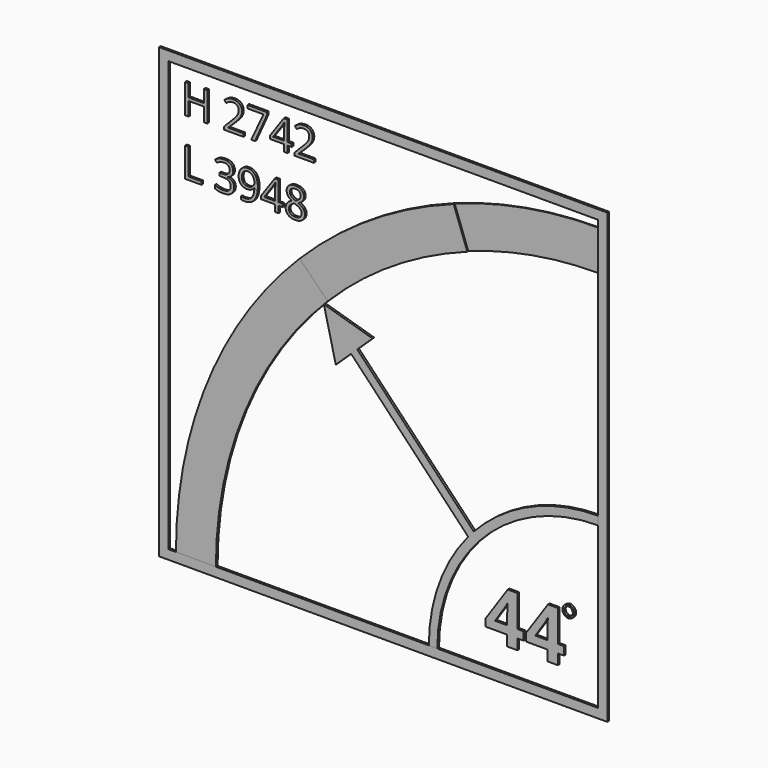
from build123d import *

# Parameters (mm, degrees)
F1_DEPTH       = 0.5
F3_DEPTH       = 0.5
F5_DEPTH       = 0.2
F6_W           = 106
F6_H           = 106
F6_W_2         = 101.6
F6_H_2         = 101.6
F7_DEPTH       = 0.5
F8_R           = 1.428350153
F8_R_2         = 1.0395037254
F8_TEXT_SIZE   = 16.6666666667
F8_TEXT_SIZE_2 = 9.7222222222
F9_DEPTH       = 0.5


# Not quite as in the source:
# - Text() gives the source's letters only with a copy of the font that has no kerning and outlines rounded to 1/6400 em; it was checked with that copy


with BuildPart() as f1:
    # F0 (on Front) → F1 (new body)
    with BuildSketch(Plane.XZ):
        with BuildLine():
            ThreePointArc((-19.7674013949, 19.7674013949), (-41.4007531902, -12.6091975676), (-48.9973761141, -50.8))
            Line((-48.9973761141, -50.8), (-39.5521000028, -50.8))
            ThreePointArc((-39.5521000028, -50.8), (-32.674455912, -16.2237482495), (-13.0885826064, 13.0885826064))
            Line((-13.0885826064, 13.0885826064), (-19.7674013949, 19.7674013949))
        make_face()
    extrude(amount=F1_DEPTH)


with BuildPart() as f3:
    # F2 (on Front) → F3 (new body)
    with BuildSketch(Plane.XZ):
        with BuildLine():
            ThreePointArc((16.6672871179, 42.9788579082), (-2.8210911002, 33.3682533292), (-19.7674013949, 19.7674013949))
            Line((-19.7674013949, 19.7674013949), (-13.0885826064, 13.0885826064))
            ThreePointArc((-13.0885826064, 13.0885826064), (2.2538520552, 25.4021882536), (19.8977618073, 34.1032016451))
            Line((19.8977618073, 34.1032016451), (16.6672871179, 42.9788579082))
        make_face()
    extrude(amount=F3_DEPTH)


with BuildPart() as f5:
    # F4 (on Front) → F5 (new body)
    with BuildSketch(Plane.XZ):
        with BuildLine():
            ThreePointArc((50.8, 48.9973761141), (33.4703675018, 47.4812297275), (16.6672871179, 42.9788579082))
            Line((16.6672871179, 42.9788579082), (19.8977960102, 34.1031076732))
            ThreePointArc((19.8977960102, 34.1031076732), (35.1105398514, 38.1793501002), (50.8, 39.552))
            Line((50.8, 39.552), (50.8, 48.9973761141))
        make_face()
    extrude(amount=F5_DEPTH)


with BuildPart() as f7:
    # F6 (on Front) → F7 (new body)
    with BuildSketch(Plane.XZ):
        Rectangle(F6_W, F6_H)
        Rectangle(F6_W_2, F6_H_2, mode=Mode.SUBTRACT)
    extrude(amount=F7_DEPTH)


with BuildPart() as f9:
    # F8 (on Front) → F9 (new body)
    with BuildSketch(Plane.XZ):
        with BuildLine():
            Line((21.4240073654, -23.6513157458), (-6.1287743468, 5.3071468295))
            Line((-6.1287743468, 5.3071468295), (-2.5064167724, 8.7536705278))
            Line((-2.5064167724, 8.7536705278), (-14.0167108476, 12.1467709243))
            Line((-14.0167108476, 12.1467709243), (-11.200074951, 0.4820136519))
            Line((-11.200074951, 0.4820136519), (-7.5777173766, 3.9285373502))
            Line((-7.5777173766, 3.9285373502), (20.098580007, -25.1597423879))
            ThreePointArc((20.098580007, -25.1597423879), (20.7518267654, -24.3972106538), (21.4240073654, -23.6513157458))
        make_face()
        with BuildLine():
            ThreePointArc((50.8, -10.8), (34.7679597394, -14.1533946308), (21.4240073654, -23.6513157458))
            ThreePointArc((21.4240073654, -23.6513157458), (20.7518267654, -24.3972106538), (20.098580007, -25.1597423879))
            ThreePointArc((20.098580007, -25.1597423879), (13.1964310223, -37.1628595321), (10.8, -50.8))
            Line((10.8, -50.8), (12.8, -50.8))
            ThreePointArc((12.8, -50.8), (23.9299423149, -23.9299423149), (50.8, -12.8))
            Line((50.8, -12.8), (50.8, -10.8))
        make_face()
        with Locations((43.8, -33)):
            Circle(F8_R)
        with Locations((43.8, -33)):
            Circle(F8_R_2, mode=Mode.SUBTRACT)
        with Locations((23.9536458333, -45)):
            Text('44', F8_TEXT_SIZE, font='Open Sans', font_style=FontStyle.BOLD, text_align=(TextAlign.LEFT, TextAlign.BOTTOM))
        with Locations((-47.8, 40.8)):
            Text('H 2742', F8_TEXT_SIZE_2, font='Open Sans', text_align=(TextAlign.LEFT, TextAlign.BOTTOM))
        with Locations((-47.8, 27.5777777778)):
            Text('L 3948', F8_TEXT_SIZE_2, font='Open Sans', text_align=(TextAlign.LEFT, TextAlign.BOTTOM))
    extrude(amount=F9_DEPTH)


solid = Compound([f1.part, f3.part, f5.part, f7.part, f9.part])
